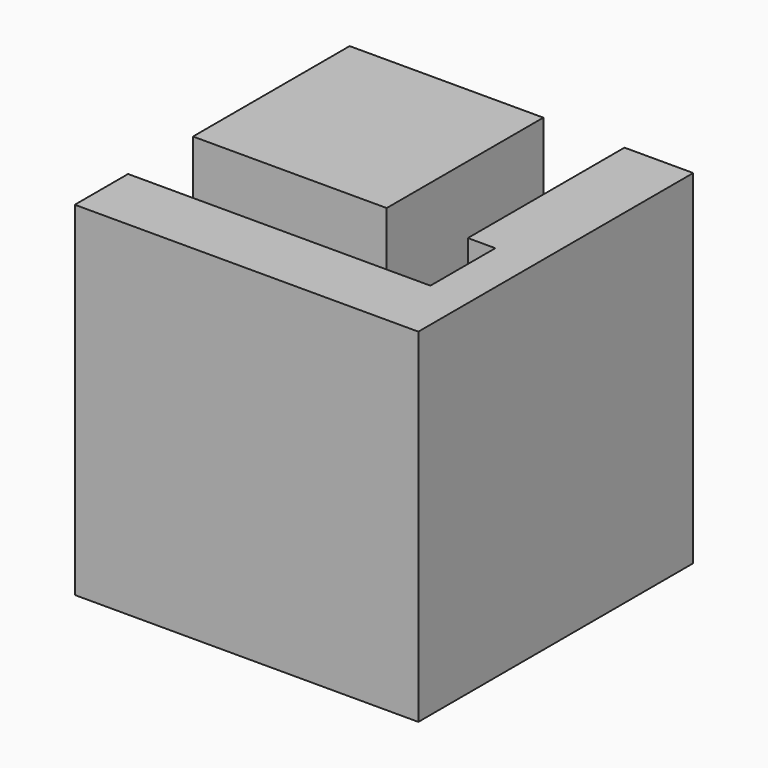
from build123d import *

# Parameters (mm, degrees)
F0_W     = 7.16
F0_H     = 7.2381474632
F1_DEPTH = 10.16
F2_W     = 7.16
F2_H     = 7.2381474632
F3_DEPTH = 2.54


# Not quite as in the source:
# - a feature of the source that left no trace in its solid (it failed there, or was rolled back) is left out


with BuildPart() as f1:
    # F0 (on Top) → F1 (new body)
    with BuildSketch(Plane.XY):
        with Locations((-5.8439813066, -2.7033329925)):
            Rectangle(F0_W, F0_H)
    extrude(amount=F1_DEPTH)



with BuildPart() as f1b:
    # F0 (on Top) → F1, piece 2 (new body)
    with BuildSketch(Plane.XY):
        Polygon((-12.4239813066, 0.9157407391), (-14.9639813066, 0.9157407391), (-14.9639813066, -11.7842592609), (-2.2639813066, -11.7842592609), (-2.2639813066, -9.3224067241), (-9.4239813066, -9.3224067241), (-12.4239813066, -9.3224067241), (-13.4399813066, -9.3224067241), (-13.4399813066, -6.3224067241), (-12.4239813066, -6.3224067241), align=None)
    extrude(amount=F1_DEPTH)


with BuildPart() as f1_1:
    add(f1.part)

    add(f1b.part)  # F3 merges F1b
    # F2 (on face) → F3 (join)
    with BuildSketch(Plane(origin=(0, 0, 0), x_dir=(1, 0, 0), z_dir=(0, 0, -1))):
        with Locations((-5.8439813066, 2.7033329925)):
            Rectangle(F2_W, F2_H)
        Polygon((-2.2639813066, 9.3224067241), (-13.4399813066, 9.3224067241), (-13.4399813066, 6.3224067241), (-12.4239813066, 6.3224067241), (-12.4239813066, -0.9157407391), (-9.4239813066, -0.9157407391), (-9.4239813066, 6.3224067241), (-2.2639813066, 6.3224067241), align=None)
        Polygon((-13.4399813066, 6.3224067241), (-13.4399813066, 9.3224067241), (-2.2639813066, 9.3224067241), (-2.2639813066, 11.7842592609), (-14.9639813066, 11.7842592609), (-14.9639813066, -0.9157407391), (-12.4239813066, -0.9157407391), (-12.4239813066, 6.3224067241), align=None)
    extrude(amount=F3_DEPTH)


with BuildPart() as f5_1:
    # F5: instance of F1
    add(f1_1.part.mirror(Plane(origin=(-8.6139813066, -4.877797716, 3.5140776699), x_dir=(0, 1, 0), z_dir=(1, 0, 0))))


solid = f5_1.part
